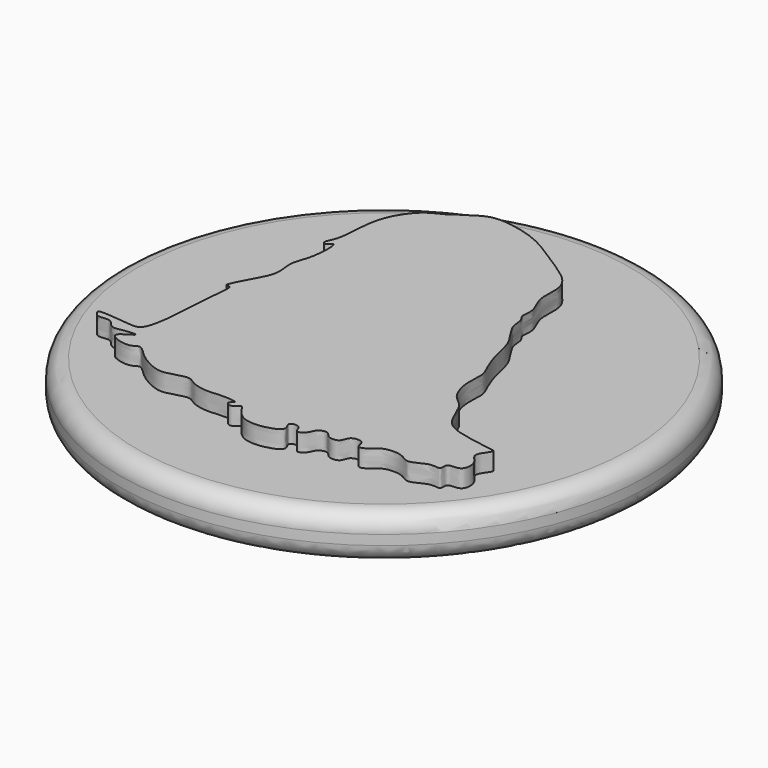
from build123d import *

# Parameters (mm, degrees)
F2_R     = 1
F5_DEPTH = 1


# Not quite as in the source:
# - a fillet or chamfer that OpenCascade refuses, or shapes differently, is made with other operations: its cross-section is extruded or revolved along the edge and cut away or added


with BuildPart() as f1:
    # F0 (on Front) → F1 (revolve)
    with BuildSketch(Plane.XZ):
        Polygon((0, 7.5), (0, 0), (4.05, 0), (4.05, 3), (6, 3), (6, 4.5), (15, 5), (15, 7.5), align=None)
    revolve(axis=Axis((0, 0, 1.9640208051), (0, 0, 1)))

    # F2
    f2_edges = [f1.edges().sort_by_distance(p)[0] for p in [
        (-15, 0, 5),
        (-15, 0, 7.5),
    ]]
    fillet(f2_edges, radius=F2_R)

    # F3: chamfer of 0.3 x 1 on 1 edges, made by hand

    # F3_s1 → F3_t2 (revolve, cut)
    with BuildSketch(Plane.XZ):
        Polygon((4.05, 1), (3.75, 0), (4.05, 0), align=None)
    revolve(axis=Axis((0, 0, 0), (0, 0, 1)), mode=Mode.SUBTRACT)

    # F4 (on face) → F5 (join)
    with BuildSketch(Plane.XY.offset(7.5)):
        with BuildLine():
            add(Edge.make_bspline(
                [(-11.4588430151, -5.8607370593), (-11.1993229963, -5.7749356022), (-9.5854029618, -6.0659980212), (-8.9697171783, -5.9267770707), (-8.6834573604, -4.667555337), (-8.6070377696, -3.0961437741), (-8.4843559593, -1.2565255187), (-8.3509531693, -0.2655123636), (-8.9062586488, -0.5223636805), (-7.9592606914, 1.0672241416), (-7.5479746186, 2.0328656575), (-7.8359187986, 3.1310745316), (-7.3090870616, 4.0502368062), (-7.2674236586, 6.0164256058), (-7.6441830084, 5.4119741942), (-7.9589824761, 5.5550416506), (-7.5857718477, 6.1548324306), (-7.509992792, 7.1646434613), (-7.4204924449, 9.0830848892), (-6.2313397977, 10.6852028918), (-5.3223426334, 10.9418087812), (-4.621566186, 11.5481438492), (-4.4659738959, 11.5679246298), (-3.6505718707, 12.2209220273), (-2.1645817788, 12.0691169433), (-0.5126177014, 11.590764582), (1.1309949383, 10.4520863161), (2.5894287848, 9.5737946598), (3.150733877, 8.6088060017), (2.881471777, 7.2589753046), (3.5972241176, 6.2783144894), (3.3400707494, 5.4823809039), (3.7315716846, 5.1925711812), (3.6148545757, 4.3971545143), (4.663020072, 3.2481481828), (4.8204713029, 1.936983178), (5.2952094143, 0.6741468641), (5.6671101761, 0.0139155322), (5.4468786749, -1.135459227), (5.9266386754, -2.4698238137), (6.7614697327, -2.832053597), (7.2029195953, -4.5410471603), (8.4192779328, -5.0613596366), (10.2913869371, -5.3302612775), (10.6918797225, -5.4048200668), (9.8661067329, -6.2516463187), (10.703266701, -6.6830970486), (10.6494386443, -7.8365468387), (9.6465633748, -7.5762760476), (9.8572714217, -8.3125321235), (9.1279854056, -8.0198398851), (8.2072816685, -8.7486426319), (7.7180953645, -8.2108852918), (6.5233026885, -8.1265788735), (5.9777493736, -8.8371473411), (5.4970119576, -8.8751237596), (5.5768818949, -8.2512476272), (4.6748045485, -8.2923320686), (4.7146060503, -8.979937847), (3.9332283283, -9.0016617769), (3.7340962678, -8.5020654339), (3.1154365919, -8.7099080729), (3.0766554484, -9.1593712072), (2.4643445668, -9.5707763775), (2.456684468, -8.8327541949), (1.6178641468, -8.9687003175), (2.1832904089, -9.5222884304), (1.3786534775, -9.9774858961), (-0.0669094107, -10.1052732481), (-0.6584763625, -9.3003552034), (-0.9105710387, -8.8937741657), (-1.2216708824, -9.4266651581), (-1.7039836956, -9.1045574344), (-1.0655964369, -8.8322601399), (-2.3059771407, -8.7517702028), (-2.9894743634, -8.8863185974), (-3.9373313573, -8.6832277167), (-4.3721033158, -8.200559899), (-5.5609396648, -8.7267579987), (-6.2835113786, -8.5597056241), (-7.2886626906, -8.0380388267), (-7.9486596958, -7.2029317029), (-8.306306253, -7.6570786432), (-9.2449631168, -7.5067976429), (-9.7557305891, -7.0654015819), (-8.4000597596, -6.4866117076), (-9.5554935119, -6.5914650176), (-10.1066079777, -6.7621027076), (-10.3956733019, -6.3791683702), (-10.6840407877, -6.13538562), (-11.2700966996, -6.3398387176), (-11.4786454536, -6.023748186), (-11.5552205259, -5.9558793432), (-11.5250992735, -5.8826424349), (-11.4588430151, -5.8607370593)],
                knots=[0, 0, 0, 0, 0.0165974467, 0.0260981134, 0.0390128174, 0.0549267526, 0.0722335107, 0.0826452505, 0.0879255099, 0.1026421053, 0.1162349489, 0.1282515919, 0.1418155809, 0.1564729905, 0.1633451284, 0.1687156796, 0.1779106159, 0.1904463039, 0.2075108647, 0.2242780504, 0.2364197653, 0.2475536608, 0.2523885148, 0.2640094257, 0.2789265415, 0.2950584232, 0.3125385308, 0.3284314234, 0.3407736006, 0.3547123536, 0.3678610933, 0.378158334, 0.3856994185, 0.3959264944, 0.4108027933, 0.4251373083, 0.4391804508, 0.4495900432, 0.4626261598, 0.4767038826, 0.4879924724, 0.503292275, 0.5175624772, 0.5344441265, 0.5398707136, 0.5509532652, 0.5614589241, 0.5725862813, 0.5825814352, 0.5902193171, 0.5991797922, 0.6116563744, 0.6211309281, 0.633900326, 0.6452732664, 0.6520381374, 0.6600553331, 0.6696246365, 0.6784602951, 0.6877337506, 0.6959201388, 0.704376225, 0.712693644, 0.7211598589, 0.7295647416, 0.7380511101, 0.7461771922, 0.7563807963, 0.7710216306, 0.7829280675, 0.7897516261, 0.7978662512, 0.8047657789, 0.8112865359, 0.8224301833, 0.8339059967, 0.8454168344, 0.8546748686, 0.8678202367, 0.8784250245, 0.8916771264, 0.9031758816, 0.9108547351, 0.9227373879, 0.9305321907, 0.9416568346, 0.9513987456, 0.9611565921, 0.9689281381, 0.9762016056, 0.985246517, 0.9921559847, 0.9957626209, 1, 1, 1, 1], degree=3))
        make_face()
    extrude(amount=F5_DEPTH)


solid = f1.part
